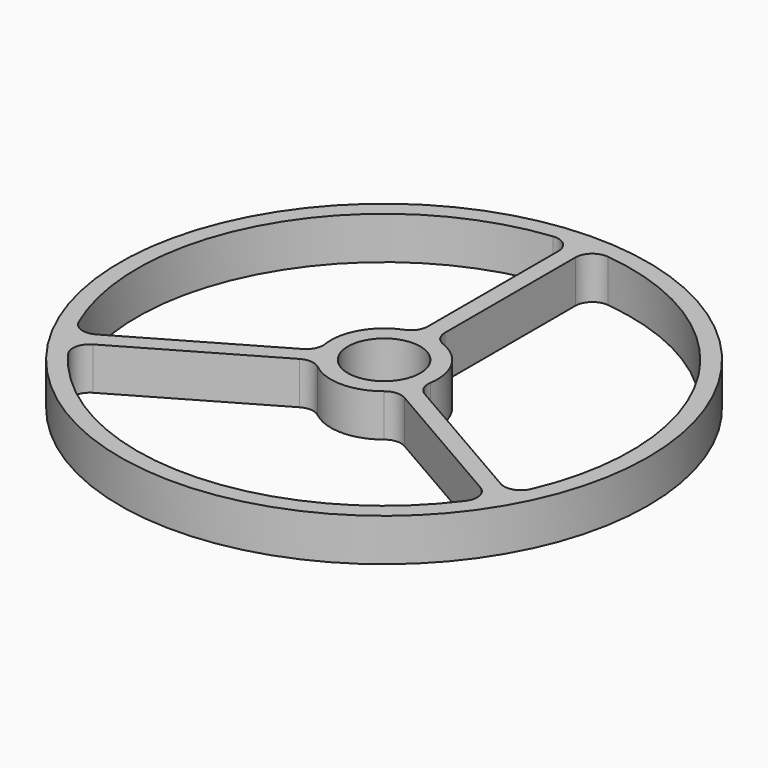
from build123d import *

# Parameters (mm, degrees)
F0_R            = 31
F0_R_2          = 4.25
F1_DEPTH        = 5
F3_DEPTH        = 25
F3_COPIES_COUNT = 3
F4_R            = 2


# Not quite as in the source:
# - a pattern or mirror of a feature is missing from the dataset's text; its kind, count and spacing are read off the source's solid


with BuildPart() as f1:
    # F0 (on Top) → F1 (new body)
    with BuildSketch(Plane.XY):
        Circle(F0_R)
        Circle(F0_R_2, mode=Mode.SUBTRACT)
    extrude(amount=F1_DEPTH)

    # F2 (on face) → F3 (cut)
    with BuildSketch(Plane.XY.offset(5)):
        with BuildLine():
            ThreePointArc((1, 6.1694813396), (5.4126587737, 3.125), (5.8429275683, -2.218715266))
            Line((5.8429275683, -2.218715266), (25.599800796, -13.6253513424))
            ThreePointArc((25.599800796, -13.6253513424), (25.1147367097, 14.5), (1, 28.9827534924))
            Line((1, 28.9827534924), (1, 6.1694813396))
        make_face()
    f3 = extrude(amount=-F3_DEPTH, mode=Mode.SUBTRACT)

    # F3_copies: F3 ×3 about axis
    f3_copies_axis = Axis((0, 0, 0), (0, 0, 1))
    for i in range(1, F3_COPIES_COUNT):
        add(f3.rotate(f3_copies_axis, i * 360 / F3_COPIES_COUNT), mode=Mode.SUBTRACT)

    # F4
    f4_edges = [f1.edges().sort_by_distance(p)[0] for p in [
        (1, 6.169481, 2.5),
        (5.842928, -2.218715, 2.5),
        (25.599801, -13.625351, 2.5),
        (1, 28.982753, 2.5),
        (24.599801, -15.357402, 2.5),
        (-24.599801, -15.357402, 2.5),
        (4.842928, -3.950766, 2.5),
        (-4.842928, -3.950766, 2.5),
        (-25.599801, -13.625351, 2.5),
        (-1, 28.982753, 2.5),
        (-1, 6.169481, 2.5),
        (-5.842928, -2.218715, 2.5),
    ]]
    fillet(f4_edges, radius=F4_R)


solid = f1.part
